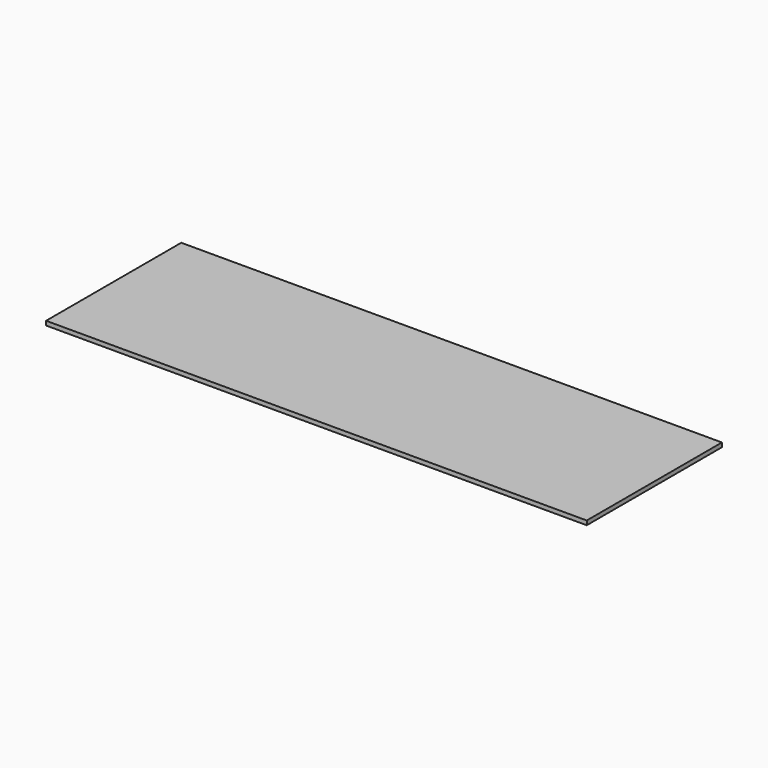
from build123d import *

# Parameters (mm, degrees)
F0_W     = 2438.4
F0_H     = 762
F5_DEPTH = 19.05


# Not quite as in the source:
# - the program builds the solid bodies; features that only make, move or delete a surface that nothing else refers to are left out


with BuildPart() as f5:
    # F0 (on Top) → F5 (new body)
    with BuildSketch(Plane.XY):
        with Locations((-2040.03204422, 3733.8)):
            Rectangle(F0_W, F0_H)
    extrude(amount=F5_DEPTH)


solid = f5.part
